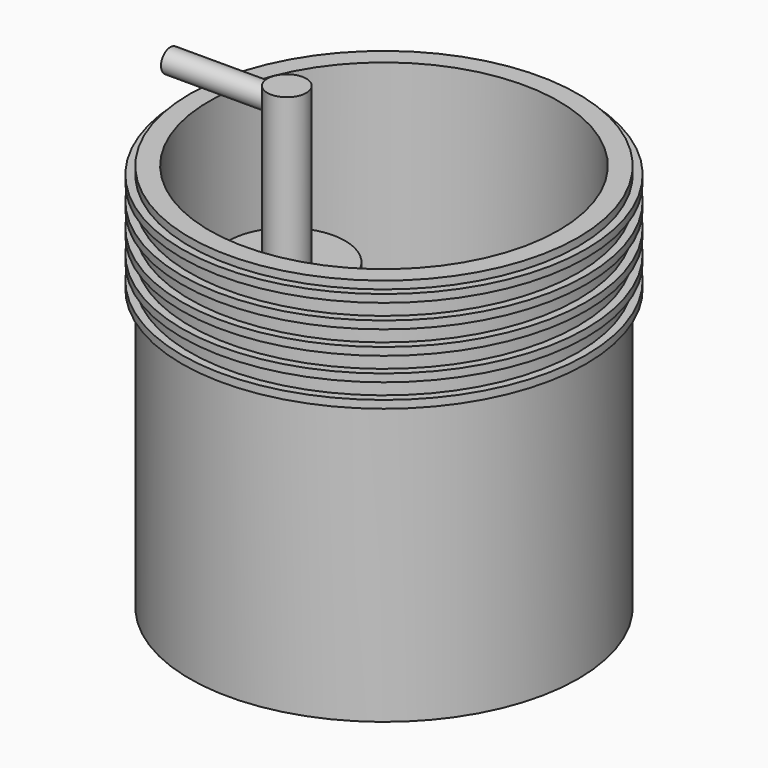
from build123d import *

# Parameters (mm, degrees)
F0_R          = 25
F1_DEPTH      = 50
F2_T          = -2.5
F3_W          = 1
F3_H          = 1
F6_START      = 2.5
F5_R          = 7.5
F6_DEPTH      = 32.5
F7_R          = 2.5
F8_DEPTH      = 20
F8_DEPTH_BACK = 1
F11_R         = 1.5
F12_DEPTH     = 15


with BuildPart() as f1:
    # F0 (on Top) → F1 (new body)
    with BuildSketch(Plane.XY):
        Circle(F0_R)
    extrude(amount=F1_DEPTH)

    # F2
    f2_openings = [f1.faces().sort_by_distance(p)[0] for p in [
        (0, 0, 50),
    ]]
    offset(amount=F2_T, openings=f2_openings)

    # F3 (on Front) → F4 (revolve)
    with BuildSketch(Plane.XZ):
        with Locations((25.5, 48.5)):
            Rectangle(F3_W, F3_H)
        with Locations((25.5, 36.5)):
            Rectangle(F3_W, F3_H)
        with Locations((25.5, 39.5)):
            Rectangle(F3_W, F3_H)
        with Locations((25.5, 42.5)):
            Rectangle(F3_W, F3_H)
        with Locations((25.5, 45.5)):
            Rectangle(F3_W, F3_H)
    revolve(axis=Axis((0, 0, 25), (0, 0, 1)))


with BuildPart() as f6:
    # F5 (on Top) → F6 (new body)
    with BuildSketch(Plane.XY.offset(F6_START)):
        with Locations((-12.5, 0)):
            Circle(F5_R)
    extrude(amount=F6_DEPTH)


with BuildPart() as f8:
    # F7 (on face) → F8 (new body, two sides)
    with BuildSketch(Plane.XY.offset(35)) as f8_sk:
        with Locations((-12.5, 0)):
            Circle(F7_R)
    extrude(amount=F8_DEPTH)
    extrude(f8_sk.sketch, amount=-F8_DEPTH_BACK)


with BuildPart() as f6_1:
    add(f6.part)

    # F9: cut F8
    add(f8.part, mode=Mode.SUBTRACT)


with BuildPart() as f8_1:
    add(f8.part)

    # F11 (on offset) → F12 (join)
    with BuildSketch(Plane.YZ.offset(-12.5)):
        with Locations((0, 53)):
            Circle(F11_R)
    extrude(amount=-F12_DEPTH)


solid = Compound([f1.part, f6_1.part, f8_1.part])
